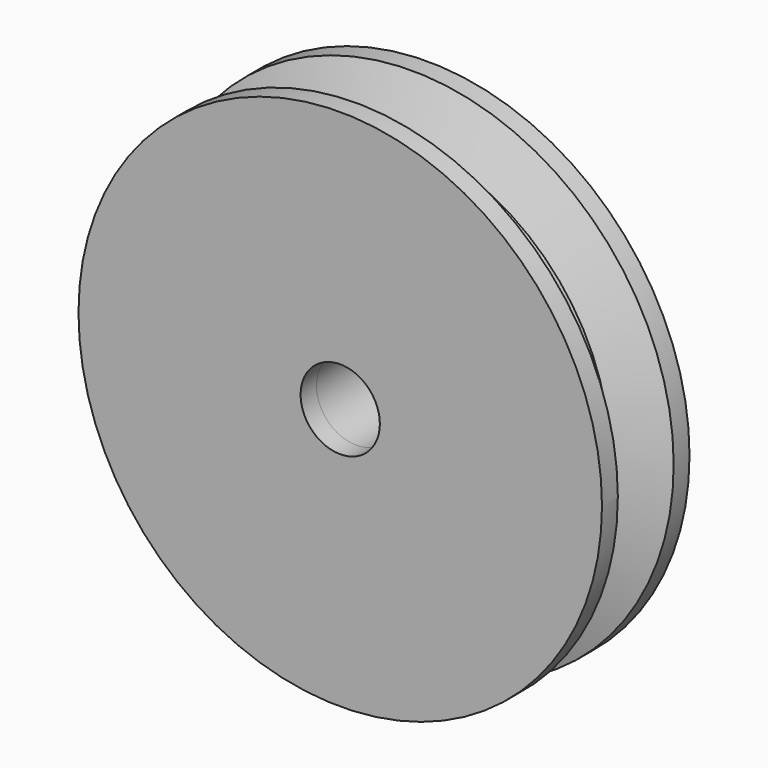
from build123d import *
from build123d import SkipClean  # not in build123d's __all__

# Parameters (mm, degrees)
F2_FACE_R    = 83.9113721036
F2_FACE_R_2  = 12.7043497663
F3_DEPTH     = 6.35
F2_FACE1_R   = 83.9113721036
F2_FACE1_R_2 = 12.7043497663
F4_DEPTH     = 6.35
F5_R         = 22.8643497663
F5_R_2       = 12.7043497663
F6_DEPTH     = 38.1
F8_D         = 5.1054
F8_DEPTH     = 84.2447919947


# Not quite as in the source:
# - after a boolean that leaves OpenCascade's solid faulty, fix() repairs it


with BuildPart() as f2:
    # F0 (on Top) → F2 (revolve)
    with BuildSketch(Plane.XY):
        Polygon((71.2107136504, 12.2464282371), (0, 12.2464282371), (0, -10.1297611803), (71.2107136504, -10.1297611803), (55.7892807321, -3.7797611803), (55.7892807321, 5.8964282371), align=None)
    revolve(axis=Axis((-12.7, 0, -0.3324198911), (0, -1, 0)))

    # F2_face (on face) → F3 (join)
    with BuildSketch(Plane(origin=(-12.7, 12.2464282371, -0.3324198911), x_dir=(-1, 0, 0), z_dir=(0, 1, 0))):
        Circle(F2_FACE_R)
        Circle(F2_FACE_R_2, mode=Mode.SUBTRACT)
    with SkipClean():  # cleaning this boolean's faces spoils the solid; the shape is the same uncleaned
        extrude(amount=F3_DEPTH)

    # F2_face1 (on face) → F4 (join)
    with BuildSketch(Plane(origin=(-12.7, -10.1297611803, -0.3324198911), x_dir=(1, 0, 0), z_dir=(0, -1, 0))):
        Circle(F2_FACE1_R)
        Circle(F2_FACE1_R_2, mode=Mode.SUBTRACT)
    extrude(amount=F4_DEPTH)

    add(f2.part.fix(), mode=Mode.REPLACE)

    # F5 (on face) → F6 (join)
    with BuildSketch(Plane(origin=(0, 18.5964282371, 0), x_dir=(-1, 0, 0), z_dir=(0, 1, 0))):
        with Locations((12.7, -0.3324198911)):
            Circle(F5_R)
        with Locations((12.7, -0.3324198911)):
            Circle(F5_R_2, mode=Mode.SUBTRACT)
    extrude(amount=F6_DEPTH)

    # F8 (through all, one way)
    with BuildSketch(Plane.XY):
        with Locations((-11.8156038225, 40.2014479041)):
            Circle(F8_D / 2)
    extrude(amount=-F8_DEPTH, mode=Mode.SUBTRACT)


solid = f2.part
